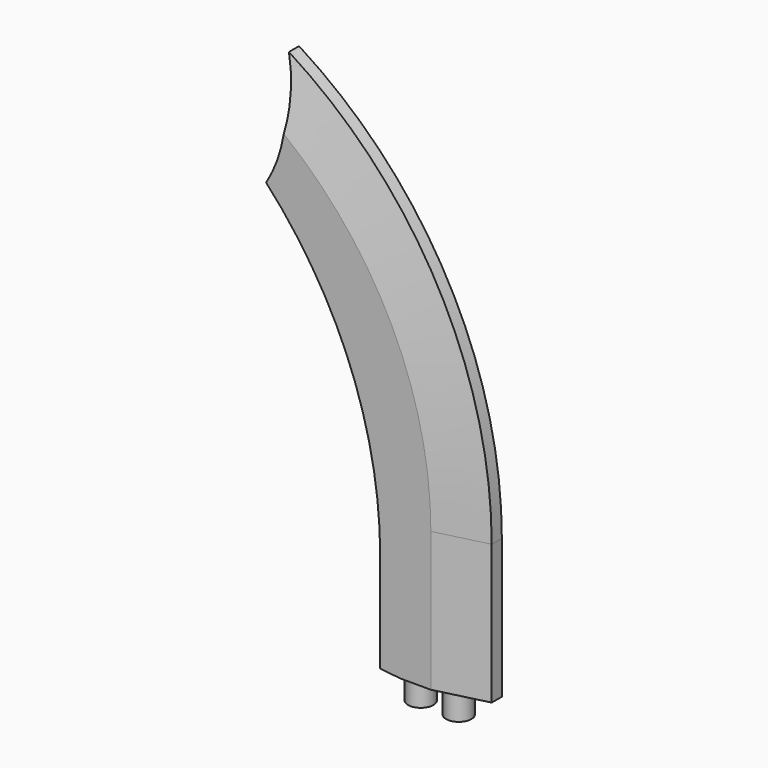
from build123d import *

# Parameters (mm, degrees)
F1_DEPTH    = 4.7625
F2_SIZE2    = 12.7
F2_SIZE     = 3.175
F3_SIZE2    = 12.7
F3_SIZE     = 3.175
F4_R        = 3.175
F5_DEPTH    = 6.35
F6_T4_DEPTH = 35.9361512716
F6_S5_R     = 3.175
F6_T6_DEPTH = 20


# Not quite as in the source:
# - a fillet or chamfer that OpenCascade refuses, or shapes differently, is made with other operations: its cross-section is extruded or revolved along the edge and cut away or added


with BuildPart() as f1:
    # F0 (on Front) → F1 (new body, symmetric)
    with BuildSketch(Plane.XZ):
        with BuildLine():
            ThreePointArc((-38.1, 127), (-36.6107102977, 112.3706344775), (-41.275, 98.425))
            ThreePointArc((-41.275, 98.425), (-20.0980859114, 64.6083576869), (-12.7, 25.4))
            Line((-12.7, 25.4), (-12.7, 0))
            Line((-12.7, 0), (12.7, 0))
            Line((12.7, 0), (12.7, 34.925))
            ThreePointArc((12.7, 34.925), (-0.8424942493, 87.5045721383), (-38.1, 127))
        make_face()
    extrude(amount=F1_DEPTH, both=True)

    # F2
    f2_edges = [f1.edges().sort_by_distance(p)[0] for p in [
        (-0.842494, -4.7625, 87.504572),
        (12.7, -4.7625, 17.4625),
    ]]
    chamfer(f2_edges, length=F2_SIZE, length2=F2_SIZE2)

    # F3
    f3_edges = [f1.edges().sort_by_distance(p)[0] for p in [
        (-0.842494, 4.7625, 87.504572),
    ]]
    f3_side = f1.faces().sort_by_distance((-0.842494, 1.5875, 87.504572))[0]
    chamfer(f3_edges, length=F3_SIZE, length2=F3_SIZE2, reference=f3_side)

    # F4 (on face) → F5 (join)
    with BuildSketch(Plane(origin=(0, 0, 0), x_dir=(1, 0, 0), z_dir=(0, 0, -1))):
        with Locations((-6.35, 0)):
            Circle(F4_R)
        with Locations((3.175, 0)):
            Circle(F4_R)
    extrude(amount=F5_DEPTH)

    # F6: chamfer of 0.508 x 5.08 on 1 edges, made by hand


with BuildPart() as f6_tool2:
    # F6_s3 → F6_t4 (new body)
    with BuildSketch(Plane.XZ.offset(-17.9680756358)):
        Polygon((-12.7, 0.508), (-7.62, 0), (-12.7, 0), align=None)
    extrude(amount=F6_T4_DEPTH)

    # F6_s5 → F6_t6 (cut, symmetric)
    with BuildSketch(Plane.XY.offset(0.3)):
        with Locations((-6.35, 0)):
            Circle(F6_S5_R)
    extrude(amount=F6_T6_DEPTH, both=True, mode=Mode.SUBTRACT)


with BuildPart() as f1_1:
    add(f1.part)

    # F6_t1: cut F6_tool2
    add(f6_tool2.part, mode=Mode.SUBTRACT)


solid = f1_1.part
